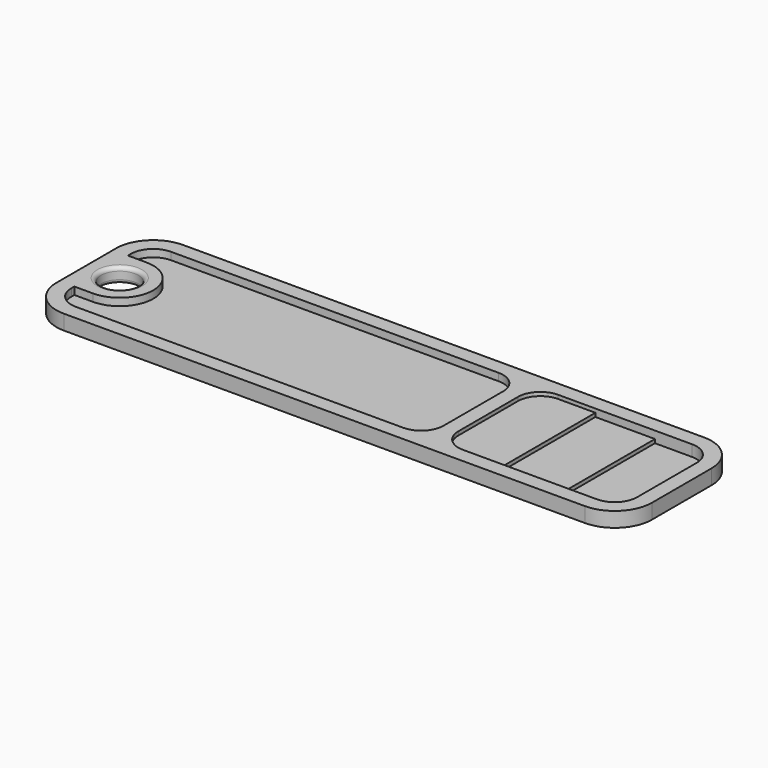
from build123d import *

# Parameters (mm, degrees)
F1_DEPTH  = 2
F3_DEPTH  = 1
F4_R      = 2.5
F5_DEPTH  = 2.001
F6_R      = 0.5
F9_DEPTH  = 1.7
F2_W      = 8
F2_H      = 16
F10_DEPTH = 1.8
F11_DEPTH = 1.9
F12_DEPTH = 0.8
F13_DEPTH = 1.2
F14_DEPTH = 1.6
F15_DEPTH = 0.5
F16_DEPTH = 1
F17_DEPTH = 1.5


with BuildPart() as f1:
    # F0 (on Top) → F1 (new body)
    with BuildSketch(Plane.XY):
        with BuildLine():
            ThreePointArc((40, 5), (38.5355339059, 8.5355339059), (35, 10))
            Line((35, 10), (-35, 10))
            ThreePointArc((-35, 10), (-38.5355339059, 8.5355339059), (-40, 5))
            Line((-40, 5), (-40, -5))
            ThreePointArc((-40, -5), (-38.5355339059, -8.5355339059), (-35, -10))
            Line((-35, -10), (35, -10))
            ThreePointArc((35, -10), (38.5355339059, -8.5355339059), (40, -5))
            Line((40, -5), (40, 5))
        make_face()
    extrude(amount=F1_DEPTH)

    # F2 (on face) → F3 (cut)
    with BuildSketch(Plane.XY.offset(2)):
        with BuildLine():
            ThreePointArc((-38, -5), (-37.1213203436, -7.1213203436), (-35, -8))
            Line((-35, -8), (9, -8))
            ThreePointArc((9, -8), (11.1213203436, -7.1213203436), (12, -5))
            Line((12, -5), (12, 5))
            ThreePointArc((12, 5), (11.1213203436, 7.1213203436), (9, 8))
            Line((9, 8), (-35, 8))
            ThreePointArc((-35, 8), (-37.1213203436, 7.1213203436), (-38, 5))
            Line((-38, 5), (-38, 4.5))
            Line((-38, 4.5), (-35.5, 4.5))
            ThreePointArc((-35.5, 4.5), (-31, 0), (-35.5, -4.5))
            Line((-35.5, -4.5), (-38, -4.5))
            Line((-38, -4.5), (-38, -5))
        make_face()
    extrude(amount=-F3_DEPTH, mode=Mode.SUBTRACT)

    # F4 (on face) → F5 (cut, through all)
    with BuildSketch(Plane.XY.offset(2)):
        with Locations((-35.5, 0)):
            Circle(F4_R)
    extrude(amount=-F5_DEPTH, mode=Mode.SUBTRACT)

    # F6
    f6_edges = [f1.edges().sort_by_distance(p)[0] for p in [
        (-38, 0, 2),
        (-38, 0, 0),
    ]]
    fillet(f6_edges, radius=F6_R)


with BuildPart() as f7_1:
    # F7: copy of F1
    add(f1.part)

    # F2 (on face) → F12 (cut, through all)
    with BuildSketch(Plane.XY.offset(2)):
        with BuildLine():
            Line((17, -8), (22, -8))
            Line((22, -8), (22, 8))
            Line((22, 8), (17, 8))
            ThreePointArc((17, 8), (14.8786796564, 7.1213203436), (14, 5))
            Line((14, 5), (14, -5))
            ThreePointArc((14, -5), (14.8786796564, -7.1213203436), (17, -8))
        make_face()
    extrude(amount=-F12_DEPTH, mode=Mode.SUBTRACT)

    # F2 (on face) → F13 (cut, through all)
    with BuildSketch(Plane.XY.offset(2)):
        with Locations((26, 0)):
            Rectangle(F2_W, F2_H)
    extrude(amount=-F13_DEPTH, mode=Mode.SUBTRACT)

    # F2 (on face) → F14 (cut, through all)
    with BuildSketch(Plane.XY.offset(2)):
        with BuildLine():
            ThreePointArc((35, -8), (37.1213203436, -7.1213203436), (38, -5))
            Line((38, -5), (38, 5))
            ThreePointArc((38, 5), (37.1213203436, 7.1213203436), (35, 8))
            Line((35, 8), (30, 8))
            Line((30, 8), (30, -8))
            Line((30, -8), (35, -8))
        make_face()
    extrude(amount=-F14_DEPTH, mode=Mode.SUBTRACT)


with BuildPart() as f8_1:
    # F8: copy of F1
    add(f1.part)

    # F2 (on face) → F9 (cut, through all)
    with BuildSketch(Plane.XY.offset(2)):
        with BuildLine():
            Line((17, -8), (22, -8))
            Line((22, -8), (22, 8))
            Line((22, 8), (17, 8))
            ThreePointArc((17, 8), (14.8786796564, 7.1213203436), (14, 5))
            Line((14, 5), (14, -5))
            ThreePointArc((14, -5), (14.8786796564, -7.1213203436), (17, -8))
        make_face()
    extrude(amount=-F9_DEPTH, mode=Mode.SUBTRACT)

    # F2 (on face) → F10 (cut, through all)
    with BuildSketch(Plane.XY.offset(2)):
        with Locations((26, 0)):
            Rectangle(F2_W, F2_H)
    extrude(amount=-F10_DEPTH, mode=Mode.SUBTRACT)

    # F2 (on face) → F11 (cut, through all)
    with BuildSketch(Plane.XY.offset(2)):
        with BuildLine():
            ThreePointArc((35, -8), (37.1213203436, -7.1213203436), (38, -5))
            Line((38, -5), (38, 5))
            ThreePointArc((38, 5), (37.1213203436, 7.1213203436), (35, 8))
            Line((35, 8), (30, 8))
            Line((30, 8), (30, -8))
            Line((30, -8), (35, -8))
        make_face()
    extrude(amount=-F11_DEPTH, mode=Mode.SUBTRACT)


with BuildPart() as f1_1:
    add(f1.part)

    # F2 (on face) → F15 (cut, through all)
    with BuildSketch(Plane.XY.offset(2)):
        with BuildLine():
            Line((17, -8), (22, -8))
            Line((22, -8), (22, 8))
            Line((22, 8), (17, 8))
            ThreePointArc((17, 8), (14.8786796564, 7.1213203436), (14, 5))
            Line((14, 5), (14, -5))
            ThreePointArc((14, -5), (14.8786796564, -7.1213203436), (17, -8))
        make_face()
    extrude(amount=-F15_DEPTH, mode=Mode.SUBTRACT)

    # F2 (on face) → F16 (cut, through all)
    with BuildSketch(Plane.XY.offset(2)):
        with Locations((26, 0)):
            Rectangle(F2_W, F2_H)
    extrude(amount=-F16_DEPTH, mode=Mode.SUBTRACT)

    # F2 (on face) → F17 (cut, through all)
    with BuildSketch(Plane.XY.offset(2)):
        with BuildLine():
            ThreePointArc((35, -8), (37.1213203436, -7.1213203436), (38, -5))
            Line((38, -5), (38, 5))
            ThreePointArc((38, 5), (37.1213203436, 7.1213203436), (35, 8))
            Line((35, 8), (30, 8))
            Line((30, 8), (30, -8))
            Line((30, -8), (35, -8))
        make_face()
    extrude(amount=-F17_DEPTH, mode=Mode.SUBTRACT)


solid = Compound([f7_1.part, f8_1.part, f1_1.part])
